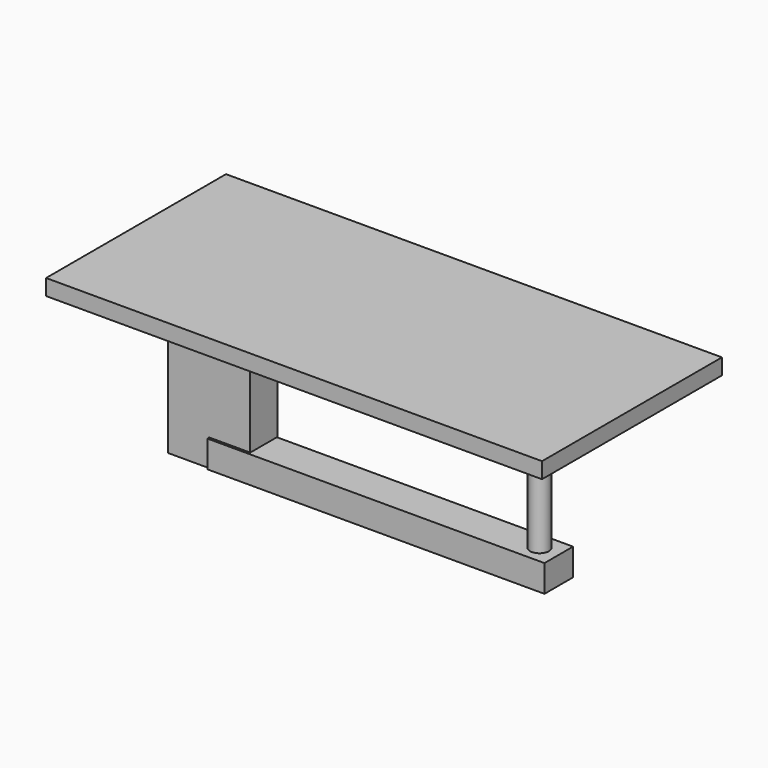
from build123d import *

# Parameters (mm, degrees)
F0_W     = 89.621424675
F0_H     = 36.9273871183
F1_DEPTH = 174.3299812078
F3_W     = 541.3100868464
F3_H     = 245.468556881
F4_DEPTH = 17.3550322652
F2_W     = 38.959980011
F2_H     = 29.5604169369
F5_DEPTH = 368.040561676
F6_R     = 10.2494359016
F7_DEPTH = 180.2812367678


with BuildPart() as f1:
    # F0 (on Top) → F1 (new body)
    with BuildSketch(Plane.XY):
        with Locations((0, 18.4636935592)):
            Rectangle(F0_W, F0_H)
    extrude(amount=F1_DEPTH)

    # F3 (on face) → F4 (join)
    with BuildSketch(Plane.XY.offset(174.3299812078)):
        with Locations((172.7937683463, 22.5193798542)):
            Rectangle(F3_W, F3_H)
    extrude(amount=F4_DEPTH)

    # F2 (on Right) → F5 (join)
    with BuildSketch(Plane.YZ):
        with Locations((16.8825984001, 14.7802084684)):
            Rectangle(F2_W, F2_H)
    extrude(amount=F5_DEPTH)

    # F6 (on face) → F7 (join)
    with BuildSketch(Plane(origin=(0, 0, 0), x_dir=(1, 0, 0), z_dir=(0, 0, -1))):
        with Locations((347.0340669155, -16.8822109699)):
            Circle(F6_R)
    extrude(amount=-F7_DEPTH)


solid = f1.part
